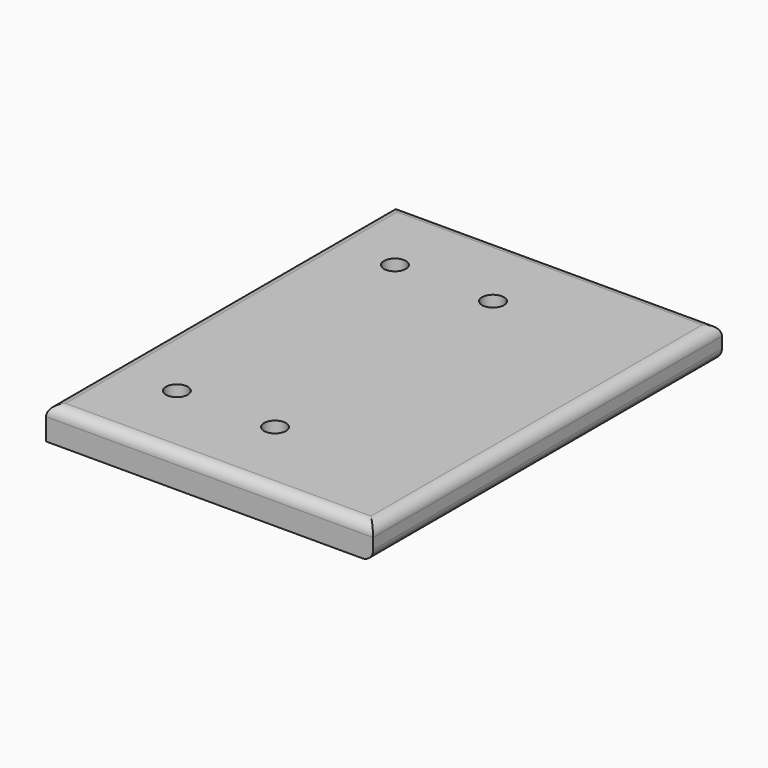
from build123d import *

# Parameters (mm, degrees)
F0_W     = 30
F0_H     = 40
F0_R     = 1
F1_DEPTH = 3
F2_R     = 1


# Not quite as in the source:
# - a feature names something its author has since deleted; it is built from what else it names


with BuildPart() as f1:
    # F0 (on Top) → F1 (new body)
    with BuildSketch(Plane.XY):
        Rectangle(F0_W, F0_H)
        with Locations((-9, -12.5)):
            Circle(F0_R, mode=Mode.SUBTRACT)
        with Locations((0, -12.5)):
            Circle(F0_R, mode=Mode.SUBTRACT)
        with Locations((-9, 12.5)):
            Circle(F0_R, mode=Mode.SUBTRACT)
        with Locations((0, 12.5)):
            Circle(F0_R, mode=Mode.SUBTRACT)
    extrude(amount=-F1_DEPTH)

    # F2
    f2_edges = [f1.edges().sort_by_distance(p)[0] for p in [
        (-15, 0, 0),
        (0, 20, 0),
        (15, 0, 0),
        (0, -20, 0),
        (15, 0, -3),
    ]]
    fillet(f2_edges, radius=F2_R)


solid = f1.part
